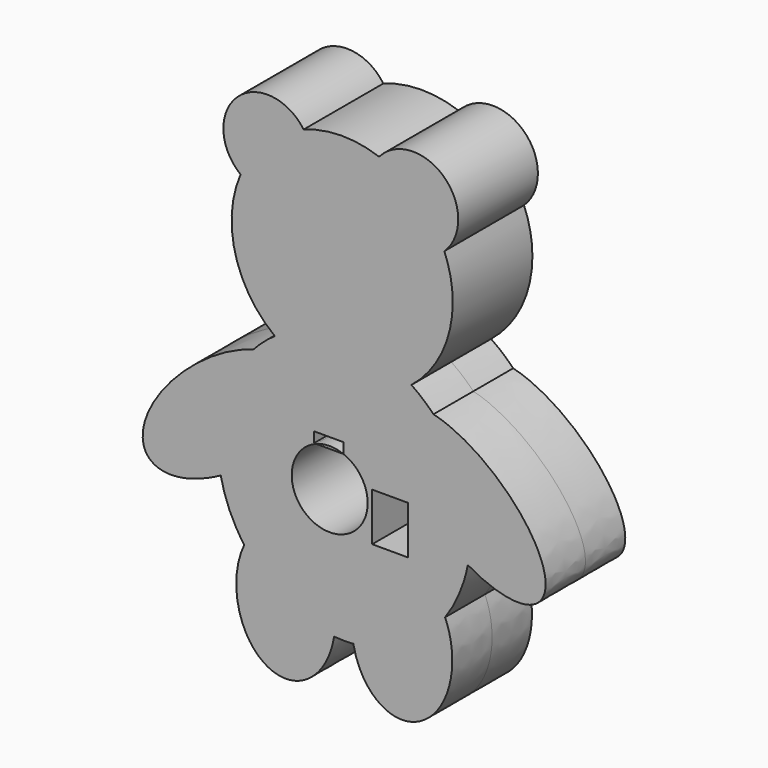
from build123d import *

# Parameters (mm, degrees)
F1_DEPTH = 12.7


with BuildPart() as f1:
    # F0 (on Front) → F1 (new body, symmetric)
    with BuildSketch(Plane.XZ):
        with BuildLine():
            ThreePointArc((21.4072020605, -0.2005026234), (29.1763847833, 9.5927644936), (31.9477205013, 21.7824314022))
            ThreePointArc((31.9477205013, 21.7824314022), (31.407623557, 27.2745103789), (29.808025642, 32.5561694654))
            ThreePointArc((29.808025642, 32.5561694654), (13.9560593574, 32.5213958074), (13.178397571, 48.3543136194))
            ThreePointArc((13.178397571, 48.3543136194), (3.538752003, 49.9752850855), (-6.075013926, 48.2072862636))
            ThreePointArc((-6.075013926, 48.2072862636), (-4.5821594527, 45.1562153753), (-4.0689174459, 41.7985032545))
            ThreePointArc((-4.0689174459, 41.7985032545), (-10.3425888827, 31.7152108279), (-22.1602111332, 32.8880466238))
            ThreePointArc((-22.1602111332, 32.8880466238), (-23.5279097172, 14.6705886204), (-13.4407785602, -0.5608315546))
            add(Edge.make_bspline(
                [(21.4072020605, -0.2005026234), (3.8738448753, 11.5030083296), (-13.4407785602, -0.5608315546)],
                knots=[2.5795956317, 2.5795956317, 2.5795956317, 3.7230991014, 3.7230991014, 3.7230991014], degree=2, weights=[1, 0.8409543917, 1]))
        make_face()
        with BuildLine():
            ThreePointArc((13.178397571, 48.3543136194), (13.9560593574, 32.5213958074), (29.808025642, 32.5561694654))
            ThreePointArc((29.808025642, 32.5561694654), (23.1724221434, 42.2228318625), (13.178397571, 48.3543136194))
        make_face()
        with BuildLine():
            ThreePointArc((13.178397571, 48.3543136194), (23.1724221434, 42.2228318625), (29.808025642, 32.5561694654))
            ThreePointArc((29.808025642, 32.5561694654), (32.423912555, 36.3391968743), (33.3451540291, 40.8453565324))
            ThreePointArc((33.3451540291, 40.8453565324), (25.8701142557, 51.6050324403), (13.178397571, 48.3543136194))
        make_face()
        with BuildLine():
            add(Edge.make_bspline(
                [(27.032929556, -4.9640346513), (24.47286462, -2.2468315132), (21.4072020605, -0.2005026234)],
                knots=[2.3555291834, 2.3555291834, 2.3555291834, 2.5795956317, 2.5795956317, 2.5795956317], degree=2, weights=[1, 0.9937308397, 1]))
            ThreePointArc((21.4072020605, -0.2005026234), (4.045552476, -6.4097372456), (-13.4407785602, -0.5608315546))
            add(Edge.make_bspline(
                [(-13.4407785602, -0.5608315546), (-16.4269767093, -2.64144373), (-18.9101642422, -5.3654058694)],
                knots=[3.7230991014, 3.7230991014, 3.7230991014, 3.9441397555, 3.9441397555, 3.9441397555], degree=2, weights=[1, 0.9938988428, 1]))
            add(Edge.make_bspline(
                [(-27.220592602, -36.3314006709), (-10.5893694739, -27.0919670095), (-7.1072871664, -14.1171674007), (-3.6252048589, -1.1423677919), (-18.9101642422, -5.3654058694)],
                knots=[1.1914468438, 1.1914468438, 1.1914468438, 2.5677054181, 2.5677054181, 3.9439639925, 3.9439639925, 3.9439639925], degree=2, weights=[1, 0.7724354431, 1, 0.7724354431, 1]))
            add(Edge.make_bspline(
                [(-27.220592602, -36.3314006709), (-25.6755646838, -43.8684917338), (-21.223233788, -49.9691174456)],
                knots=[4.9263462771, 4.9263462771, 4.9263462771, 5.3708124747, 5.3708124747, 5.3708124747], degree=2, weights=[1, 0.9754076882, 1]))
            add(Edge.make_bspline(
                [(1.6894122595, -63.1094222428), (3.990089745, -49.0501097367), (-5.7417760212, -43.4689262213), (-15.4736417874, -37.887742706), (-21.223233788, -49.9691174456)],
                knots=[1.3510901139, 1.3510901139, 1.3510901139, 2.7437488102, 2.7437488102, 4.1364075066, 4.1364075066, 4.1364075066], degree=2, weights=[1, 0.7672017282, 1, 0.7672017282, 1]))
            add(Edge.make_bspline(
                [(1.6894122595, -63.1094222428), (2.9663677621, -63.2172799366), (4.2473710941, -63.2172799366)],
                knots=[6.2036673158, 6.2036673158, 6.2036673158, 6.2831853072, 6.2831853072, 6.2831853072], degree=2, weights=[1, 0.9992097152, 1]))
            add(Edge.make_bspline(
                [(4.2473710941, -63.2172799366), (5.4210318652, -63.2172799366), (6.5915787023, -63.1267179419)],
                knots=[0, 0, 0, 0.0728608894, 0.0728608894, 0.0728608894], degree=2, weights=[1, 0.9993364847, 1]))
            add(Edge.make_bspline(
                [(29.9807177647, -49.6040588443), (24.2311078692, -36.6154787146), (13.9923485543, -42.5351173737), (3.7535892394, -48.4547560328), (6.5915787023, -63.1267179419)],
                knots=[2.1142110715, 2.1142110715, 2.1142110715, 3.5423376984, 3.5423376984, 4.9704643252, 4.9704643252, 4.9704643252], degree=2, weights=[1, 0.7557070179, 1, 0.7557070179, 1]))
            add(Edge.make_bspline(
                [(29.9807177647, -49.6040588443), (34.3392330374, -43.4630345178), (35.7943407329, -35.9346430319)],
                knots=[0.9258249083, 0.9258249083, 0.9258249083, 1.3687189484, 1.3687189484, 1.3687189484], degree=2, weights=[1, 0.9755806451, 1]))
            add(Edge.make_bspline(
                [(17.4818759947, -6.6058057692), (6.8734541188, -19.0145870238), (35.7943407329, -35.9346430319)],
                knots=[0, 0, 0, 1.9426934521, 1.9426934521, 1.9426934521], degree=2, weights=[1, 0.5641881238, 1]))
            add(Edge.make_bspline(
                [(27.032929556, -4.9640346513), (20.2593941608, -3.356913921), (17.4818759947, -6.6058057692)],
                knots=[5.5513806327, 5.5513806327, 5.5513806327, 6.2831853072, 6.2831853072, 6.2831853072], degree=2, weights=[1, 0.9338012923, 1]))
        make_face()
        with BuildLine():
            ThreePointArc((7.6989617268, -23.8198920655), (9.594748521, -26.8584254178), (10.2568488529, -30.3781293333))
            ThreePointArc((10.2568488529, -30.3781293333), (-4.9042904668, -38.3689082877), (-2.9271558048, -21.3452884523))
            Line((-2.9271558048, -21.3452884523), (-3.4228879958, -21.3452884523))
            Line((-3.4228879958, -21.3452884523), (-3.4228879958, -18.6832621694))
            Line((-3.4228879958, -18.6832621694), (0, -18.6832621694))
            Line((0, -18.6832621694), (4.0681211865, -18.6832621694))
            Line((4.0681211865, -18.6832621694), (4.0681211865, -21.3452884523))
            ThreePointArc((4.0681211865, -21.3452884523), (6.0257103863, -22.3739941384), (7.6989617268, -23.8198920655))
        make_face(mode=Mode.SUBTRACT)
        Polygon((11.4096151665, -39.2205929384), (11.4096151665, -26.9552450627), (15.9734645858, -26.9552450627), (20.5373140052, -26.9552450627), (20.5373140052, -39.2205929384), align=None, mode=Mode.SUBTRACT)
        with BuildLine():
            ThreePointArc((-13.4407785602, -0.5608315546), (4.045552476, -6.4097372456), (21.4072020605, -0.2005026234))
            add(Edge.make_bspline(
                [(21.4072020605, -0.2005026234), (3.8738448753, 11.5030083296), (-13.4407785602, -0.5608315546)],
                knots=[2.5795956317, 2.5795956317, 2.5795956317, 3.7230991014, 3.7230991014, 3.7230991014], degree=2, weights=[1, 0.8409543917, 1]))
        make_face()
        with BuildLine():
            add(Edge.make_bspline(
                [(35.7943407329, -35.9346430319), (60.8095787908, -50.5697140325), (55.1097658811, -30.4215130287), (49.4099529714, -10.2733120249), (27.032929556, -4.9640346513)],
                knots=[1.9426934521, 1.9426934521, 1.9426934521, 3.7470370424, 3.7470370424, 5.5513806327, 5.5513806327, 5.5513806327], degree=2, weights=[1, 0.619907278, 1, 0.619907278, 1]))
            add(Edge.make_bspline(
                [(35.7943407329, -35.9346430319), (39.2700257665, -17.9522505972), (27.032929556, -4.9640346513)],
                knots=[1.3687189484, 1.3687189484, 1.3687189484, 2.3555291834, 2.3555291834, 2.3555291834], degree=2, weights=[1, 0.88072521, 1]))
        make_face()
        with BuildLine():
            add(Edge.make_bspline(
                [(35.7943407329, -35.9346430319), (39.2700257665, -17.9522505972), (27.032929556, -4.9640346513)],
                knots=[1.3687189484, 1.3687189484, 1.3687189484, 2.3555291834, 2.3555291834, 2.3555291834], degree=2, weights=[1, 0.88072521, 1]))
            add(Edge.make_bspline(
                [(27.032929556, -4.9640346513), (20.2593941608, -3.356913921), (17.4818759947, -6.6058057692)],
                knots=[5.5513806327, 5.5513806327, 5.5513806327, 6.2831853072, 6.2831853072, 6.2831853072], degree=2, weights=[1, 0.9338012923, 1]))
            add(Edge.make_bspline(
                [(17.4818759947, -6.6058057692), (6.8734541188, -19.0145870238), (35.7943407329, -35.9346430319)],
                knots=[0, 0, 0, 1.9426934521, 1.9426934521, 1.9426934521], degree=2, weights=[1, 0.5641881238, 1]))
        make_face()
        with BuildLine():
            ThreePointArc((-4.0689174459, 41.7985032545), (-4.5821594527, 45.1562153753), (-6.075013926, 48.2072862636))
            ThreePointArc((-6.075013926, 48.2072862636), (-15.6898722823, 42.198538731), (-22.1602111332, 32.8880466238))
            ThreePointArc((-22.1602111332, 32.8880466238), (-10.3425888827, 31.7152108279), (-4.0689174459, 41.7985032545))
        make_face()
        with BuildLine():
            ThreePointArc((-22.1602111332, 32.8880466238), (-15.6898722823, 42.198538731), (-6.075013926, 48.2072862636))
            ThreePointArc((-6.075013926, 48.2072862636), (-23.0605895831, 49.9377897728), (-22.1602111332, 32.8880466238))
        make_face()
        with BuildLine():
            add(Edge.make_bspline(
                [(-27.220592602, -36.3314006709), (-10.5893694739, -27.0919670095), (-7.1072871664, -14.1171674007), (-3.6252048589, -1.1423677919), (-18.9101642422, -5.3654058694)],
                knots=[1.1914468438, 1.1914468438, 1.1914468438, 2.5677054181, 2.5677054181, 3.9439639925, 3.9439639925, 3.9439639925], degree=2, weights=[1, 0.7724354431, 1, 0.7724354431, 1]))
            add(Edge.make_bspline(
                [(-18.9101642422, -5.3654058694), (-30.8773052041, -18.492903678), (-27.220592602, -36.3314006709)],
                knots=[3.9441397555, 3.9441397555, 3.9441397555, 4.9263462771, 4.9263462771, 4.9263462771], degree=2, weights=[1, 0.8818130986, 1]))
        make_face()
        with BuildLine():
            add(Edge.make_bspline(
                [(-18.9101642422, -5.3654058694), (-30.8773052041, -18.492903678), (-27.220592602, -36.3314006709)],
                knots=[3.9441397555, 3.9441397555, 3.9441397555, 4.9263462771, 4.9263462771, 4.9263462771], degree=2, weights=[1, 0.8818130986, 1]))
            add(Edge.make_bspline(
                [(-18.9101642422, -5.3654058694), (-62.7356726046, -17.473831279), (-45.8018668681, -38.0363134591)],
                knots=[3.9439639925, 3.9439639925, 3.9439639925, 6.2831853072, 6.2831853072, 6.2831853072], degree=2, weights=[1, 0.3905101422, 1]))
            add(Edge.make_bspline(
                [(-45.8018668681, -38.0363134591), (-40.9325572153, -43.9490476976), (-27.220592602, -36.3314006709)],
                knots=[0, 0, 0, 1.1914468438, 1.1914468438, 1.1914468438], degree=2, weights=[1, 0.8277427979, 1]))
        make_face()
        with BuildLine():
            add(Edge.make_bspline(
                [(18.9978633271, -76.1678158343), (41.7396043038, -76.1678158343), (29.9807177647, -49.6040588443)],
                knots=[0, 0, 0, 2.1142110715, 2.1142110715, 2.1142110715], degree=2, weights=[1, 0.4913950322, 1]))
            add(Edge.make_bspline(
                [(6.5915787023, -63.1267179419), (21.1844822405, -61.9977050648), (29.9807177647, -49.6040588443)],
                knots=[0.0728608894, 0.0728608894, 0.0728608894, 0.9258249083, 0.9258249083, 0.9258249083], degree=2, weights=[1, 0.9104266694, 1]))
            add(Edge.make_bspline(
                [(6.5915787023, -63.1267179419), (9.114111042, -76.1678158343), (18.9978633271, -76.1678158343)],
                knots=[4.9704643252, 4.9704643252, 4.9704643252, 6.2831853072, 6.2831853072, 6.2831853072], degree=2, weights=[1, 0.7922184388, 1]))
        make_face()
        with BuildLine():
            add(Edge.make_bspline(
                [(6.5915787023, -63.1267179419), (21.1844822405, -61.9977050648), (29.9807177647, -49.6040588443)],
                knots=[0.0728608894, 0.0728608894, 0.0728608894, 0.9258249083, 0.9258249083, 0.9258249083], degree=2, weights=[1, 0.9104266694, 1]))
            add(Edge.make_bspline(
                [(29.9807177647, -49.6040588443), (24.2311078692, -36.6154787146), (13.9923485543, -42.5351173737), (3.7535892394, -48.4547560328), (6.5915787023, -63.1267179419)],
                knots=[2.1142110715, 2.1142110715, 2.1142110715, 3.5423376984, 3.5423376984, 4.9704643252, 4.9704643252, 4.9704643252], degree=2, weights=[1, 0.7557070179, 1, 0.7557070179, 1]))
        make_face()
        with BuildLine():
            add(Edge.make_bspline(
                [(1.6894122595, -63.1094222428), (3.990089745, -49.0501097367), (-5.7417760212, -43.4689262213), (-15.4736417874, -37.887742706), (-21.223233788, -49.9691174456)],
                knots=[1.3510901139, 1.3510901139, 1.3510901139, 2.7437488102, 2.7437488102, 4.1364075066, 4.1364075066, 4.1364075066], degree=2, weights=[1, 0.7672017282, 1, 0.7672017282, 1]))
            add(Edge.make_bspline(
                [(-21.223233788, -49.9691174456), (-12.5084441764, -61.9102042206), (1.6894122595, -63.1094222428)],
                knots=[5.3708124747, 5.3708124747, 5.3708124747, 6.2036673158, 6.2036673158, 6.2036673158], degree=2, weights=[1, 0.9145398668, 1]))
        make_face()
        with BuildLine():
            add(Edge.make_bspline(
                [(-21.223233788, -49.9691174456), (-12.5084441764, -61.9102042206), (1.6894122595, -63.1094222428)],
                knots=[5.3708124747, 5.3708124747, 5.3708124747, 6.2036673158, 6.2036673158, 6.2036673158], degree=2, weights=[1, 0.9145398668, 1]))
            add(Edge.make_bspline(
                [(-21.223233788, -49.9691174456), (-33.8898636884, -76.5849716658), (-10.6337546143, -76.5849716658)],
                knots=[4.1364075066, 4.1364075066, 4.1364075066, 6.2831853072, 6.2831853072, 6.2831853072], degree=2, weights=[1, 0.4771487326, 1]))
            add(Edge.make_bspline(
                [(-10.6337546143, -76.5849716658), (-0.5157377539, -76.5849716658), (1.6894122595, -63.1094222428)],
                knots=[0, 0, 0, 1.3510901139, 1.3510901139, 1.3510901139], degree=2, weights=[1, 0.7803662306, 1]))
        make_face()
    extrude(amount=F1_DEPTH, both=True)


with BuildPart() as f1b:
    # F0 (on Front) → F1, piece 2 (new body, symmetric)
    with BuildSketch(Plane.XZ):
        with BuildLine():
            ThreePointArc((4.0681211865, -21.3452884523), (0.5704826908, -20.6917631711), (-2.9271558048, -21.3452884523))
            Line((-2.9271558048, -21.3452884523), (4.0681211865, -21.3452884523))
        make_face()
    extrude(amount=F1_DEPTH, both=True)


solid = Compound([f1.part, f1b.part])
